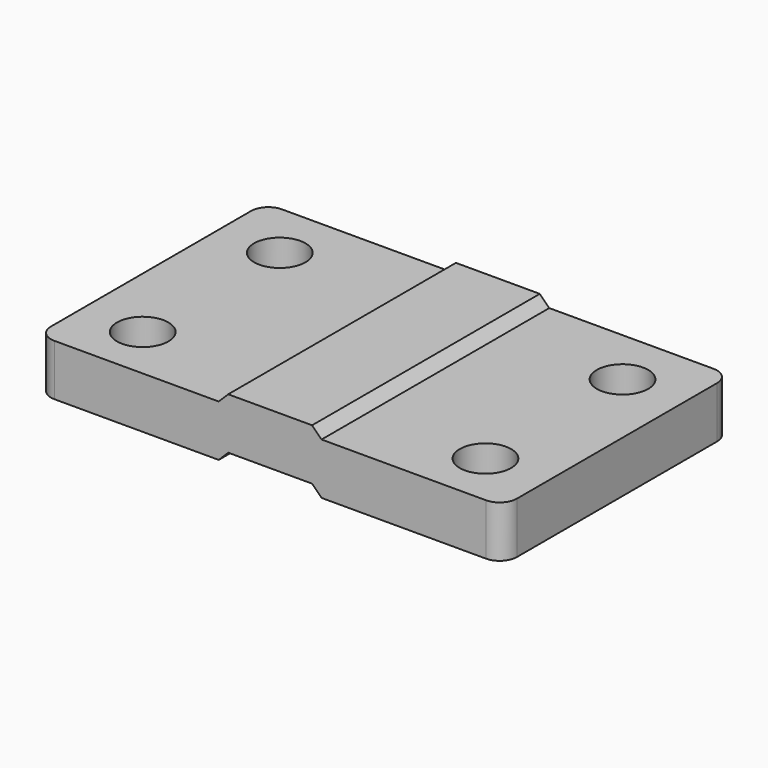
from build123d import *

# Parameters (mm, degrees)
F1_DEPTH = 15
F4_DEPTH = 83.051
F7_DEPTH = 83.05
F8_R     = 5
F10_D    = 15


with BuildPart() as f1:
    # F0 (on Top) → F1 (new body)
    with BuildSketch(Plane.XY):
        Polygon((-67.98, 0), (0, 0), (67.98, 0), (67.98, 83.05), (-67.98, 83.05), align=None)
    extrude(amount=F1_DEPTH)

    # F3 (on offset) → F4 (cut, through all)
    with BuildSketch(Plane.XZ):
        Polygon((-15, 0), (0, 0), (15, 0), (12.24, 2.76), (-12.24, 2.76), align=None)
    extrude(amount=-F4_DEPTH, mode=Mode.SUBTRACT)

    # F6 (on offset) → F7 (join)
    with BuildSketch(Plane.XZ):
        Polygon((-15, 15), (0, 15), (15, 15), (12.24, 17.76), (-12.24, 17.76), align=None)
    extrude(amount=-F7_DEPTH)

    # F8
    f8_edges = [f1.edges().sort_by_distance(p)[0] for p in [
        (-67.98, 0, 7.5),
        (67.98, 0, 7.5),
        (67.98, 83.05, 7.5),
        (-67.98, 83.05, 7.5),
    ]]
    fillet(f8_edges, radius=F8_R)

    # F10 (through all)
    with Locations(Plane(origin=(0, 0, 0), x_dir=(1, 0, 0), z_dir=(0, 0, -1))):
        with Locations((-49.98, -66), (-49.98, -16), (50.02, -66), (50.02, -16)):
            Hole(F10_D / 2)


solid = f1.part
